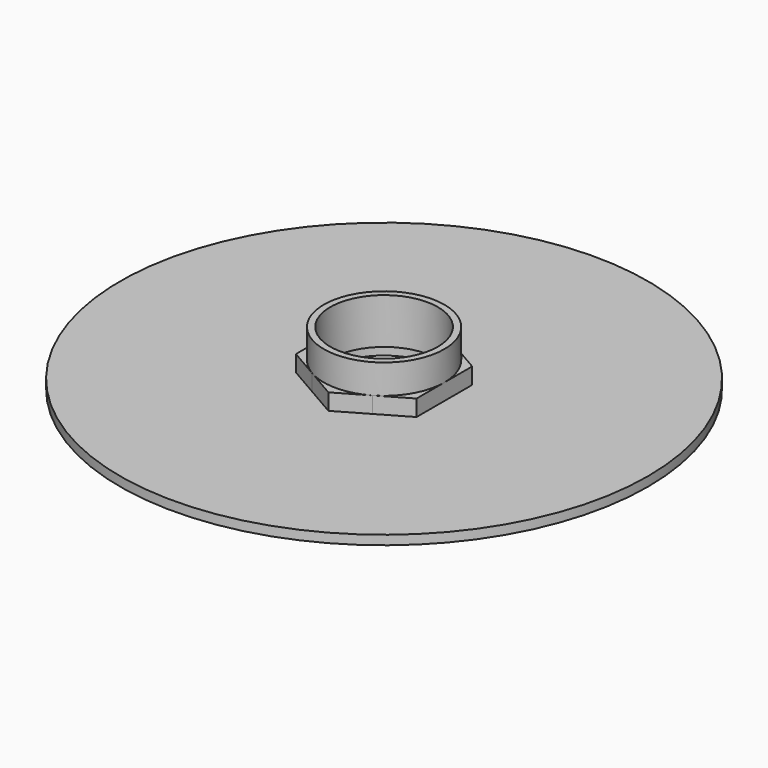
from build123d import *

# Parameters (mm, degrees)
F1_DEPTH = 5
F2_R     = 18.5
F3_DEPTH = 9
F4_R     = 16.5
F5_DEPTH = 25
F6_R     = 81
F7_DEPTH = 2.84
F8_R     = 17.4877623158
F9_DEPTH = 25


with BuildPart() as f1:
    # F0 (on Top) → F1 (new body)
    with BuildSketch(Plane.XY):
        with BuildLine():
            Line((18.5, 0), (18.5, 10.68097998))
            Line((18.5, 10.68097998), (9.2500001737, 16.0214698697))
            ThreePointArc((9.2500001737, 16.0214698697), (16.0214700202, 9.2499999131), (18.5, 0))
        make_face()
        with BuildLine():
            ThreePointArc((9.2500002367, -16.0214698334), (16.0214700383, -9.2499998817), (18.5, 0))
            ThreePointArc((18.5, 0), (16.0214700202, 9.2499999131), (9.2500001737, 16.0214698697))
            ThreePointArc((9.2500001737, 16.0214698697), (3.666e-07, 18.5), (-9.2499995387, 16.0214702364))
            ThreePointArc((-9.2499995387, 16.0214702364), (-16.0214698368, 9.2500002307), (-18.5, 0))
            ThreePointArc((-18.5, 0), (-16.0214699908, -9.2499999641), (-9.2500000719, -16.0214699285))
            ThreePointArc((-9.2500000719, -16.0214699285), (9.51e-08, -18.5), (9.2500002367, -16.0214698334))
        make_face()
        with BuildLine():
            Line((18.5, -10.68097998), (18.5, 0))
            ThreePointArc((18.5, 0), (16.0214700383, -9.2499998817), (9.2500002367, -16.0214698334))
            Line((9.2500002367, -16.0214698334), (18.5, -10.68097998))
        make_face()
        with BuildLine():
            ThreePointArc((-9.2499995387, 16.0214702364), (3.666e-07, 18.5), (9.2500001737, 16.0214698697))
            Line((9.2500001737, 16.0214698697), (0, 21.36195996))
            Line((0, 21.36195996), (-9.2499995387, 16.0214702364))
        make_face()
        with BuildLine():
            Line((0, -21.36195996), (9.2500002367, -16.0214698334))
            ThreePointArc((9.2500002367, -16.0214698334), (9.51e-08, -18.5), (-9.2500000719, -16.0214699285))
            Line((-9.2500000719, -16.0214699285), (0, -21.36195996))
        make_face()
        with BuildLine():
            ThreePointArc((-18.5, 0), (-16.0214698368, 9.2500002307), (-9.2499995387, 16.0214702364))
            Line((-9.2499995387, 16.0214702364), (-18.5, 10.68097998))
            Line((-18.5, 10.68097998), (-18.5, 0))
        make_face()
        with BuildLine():
            Line((-18.5, -10.68097998), (-9.2500000719, -16.0214699285))
            ThreePointArc((-9.2500000719, -16.0214699285), (-16.0214699908, -9.2499999641), (-18.5, 0))
            Line((-18.5, 0), (-18.5, -10.68097998))
        make_face()
    extrude(amount=F1_DEPTH)

    # F2 (on face) → F3 (join)
    with BuildSketch(Plane.XY.offset(5)):
        Circle(F2_R)
    extrude(amount=F3_DEPTH)

    # F4 (on face) → F5 (cut)
    with BuildSketch(Plane.XY.offset(14)):
        Circle(F4_R)
    extrude(amount=-F5_DEPTH, mode=Mode.SUBTRACT)

    # F6 (on Top) → F7 (join)
    with BuildSketch(Plane.XY):
        Circle(F6_R)
    extrude(amount=-F7_DEPTH)

    # F8 (on face) → F9 (cut)
    with BuildSketch(Plane.XY):
        Circle(F8_R)
    extrude(amount=-F9_DEPTH, mode=Mode.SUBTRACT)


solid = f1.part
